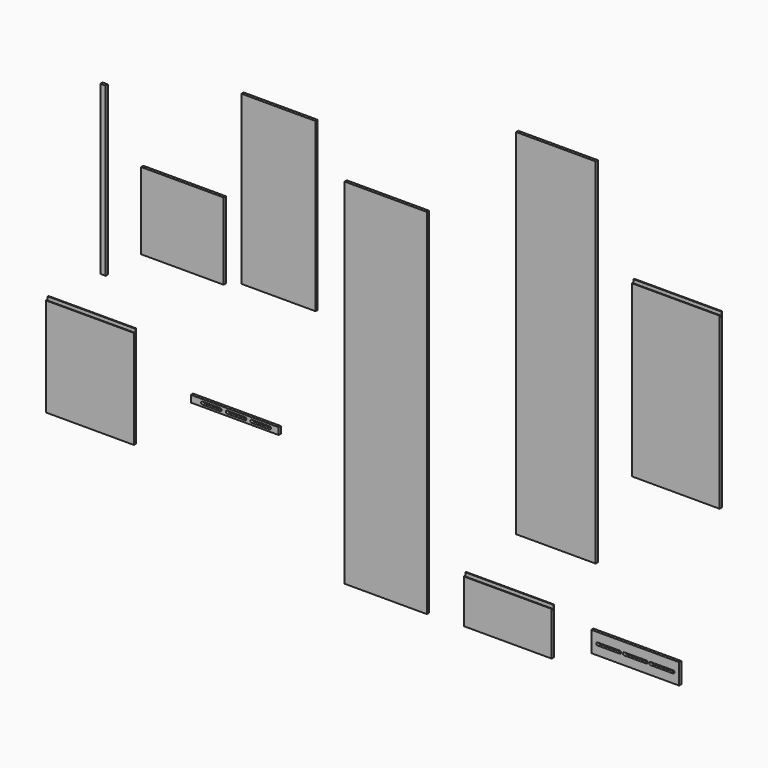
from build123d import *

# Parameters (mm, degrees)
F0_W      = 60
F0_H      = 258
F1_DEPTH  = 2
F2_W      = 58
F2_H      = 258
F3_DEPTH  = 2
F4_W      = 60
F4_H      = 56
F5_DEPTH  = 2
F6_W      = 64
F6_H      = 5
F7_DEPTH  = 2
F8_W      = 64
F8_H      = 74
F9_DEPTH  = 2
F10_W     = 64
F10_H     = 15
F11_DEPTH = 2
F13_DEPTH = 4
F14_W     = 64
F14_H     = 126
F15_DEPTH = 2
F16_W     = 64
F16_H     = 34
F17_DEPTH = 2
F18_W     = 54
F18_H     = 122
F19_DEPTH = 2
F20_W     = 4
F20_H     = 122
F21_DEPTH = 2
F23_DEPTH = 64
F24_R     = 0.2
F26_DEPTH = 64
F27_R     = 0.2
F29_DEPTH = 64
F30_R     = 0.2


with BuildPart() as f1:
    # F0 (on Front) → F1 (new body)
    with BuildSketch(Plane.XZ):
        with Locations((-45.8140162975, 94.1403650641)):
            Rectangle(F0_W, F0_H)
    extrude(amount=F1_DEPTH)


with BuildPart() as f3:
    # F2 (on Front) → F3 (new body)
    with BuildSketch(Plane.XZ):
        with Locations((78.1819216013, 166.5537835062)):
            Rectangle(F2_W, F2_H)
    extrude(amount=F3_DEPTH)


with BuildPart() as f5:
    # F4 (on Front) → F5 (new body)
    with BuildSketch(Plane.XZ):
        with Locations((-193.9391981363, 156.2652424913)):
            Rectangle(F4_W, F4_H)
    extrude(amount=F5_DEPTH)


with BuildPart() as f7:
    # F6 (on Front) → F7 (new body)
    with BuildSketch(Plane.XZ):
        with Locations((-155.7672946453, 47.4037402868)):
            Rectangle(F6_W, F6_H)
        with BuildLine():
            ThreePointArc((-180.3556742668, 47.3932959139), (-180.062781048, 48.1004026951), (-179.3556742668, 48.3932959139))
            Line((-179.3556742668, 48.3932959139), (-166.3556742668, 48.3932959139))
            ThreePointArc((-166.3556742668, 48.3932959139), (-165.6485674856, 48.1004026951), (-165.3556742668, 47.3932959139))
            ThreePointArc((-165.3556742668, 47.3932959139), (-165.6485674856, 46.6861891327), (-166.3556742668, 46.3932959139))
            Line((-166.3556742668, 46.3932959139), (-179.3556742668, 46.3932959139))
            ThreePointArc((-179.3556742668, 46.3932959139), (-180.062781048, 46.6861891327), (-180.3556742668, 47.3932959139))
        make_face(mode=Mode.SUBTRACT)
        with BuildLine():
            ThreePointArc((-162.3556742668, 47.3932959139), (-162.062781048, 48.1004026951), (-161.3556742668, 48.3932959139))
            Line((-161.3556742668, 48.3932959139), (-148.3556742668, 48.3932959139))
            ThreePointArc((-148.3556742668, 48.3932959139), (-147.6485674856, 48.1004026951), (-147.3556742668, 47.3932959139))
            ThreePointArc((-147.3556742668, 47.3932959139), (-147.6485674856, 46.6861891327), (-148.3556742668, 46.3932959139))
            Line((-148.3556742668, 46.3932959139), (-161.3556742668, 46.3932959139))
            ThreePointArc((-161.3556742668, 46.3932959139), (-162.062781048, 46.6861891327), (-162.3556742668, 47.3932959139))
        make_face(mode=Mode.SUBTRACT)
        with BuildLine():
            ThreePointArc((-144.3556742668, 47.3932959139), (-144.062781048, 48.1004026951), (-143.3556742668, 48.3932959139))
            Line((-143.3556742668, 48.3932959139), (-130.3556742668, 48.3932959139))
            ThreePointArc((-130.3556742668, 48.3932959139), (-129.6485674856, 48.1004026951), (-129.3556742668, 47.3932959139))
            ThreePointArc((-129.3556742668, 47.3932959139), (-129.6485674856, 46.6861891327), (-130.3556742668, 46.3932959139))
            Line((-130.3556742668, 46.3932959139), (-143.3556742668, 46.3932959139))
            ThreePointArc((-143.3556742668, 46.3932959139), (-144.062781048, 46.6861891327), (-144.3556742668, 47.3932959139))
        make_face(mode=Mode.SUBTRACT)
    extrude(amount=F7_DEPTH)


with BuildPart() as f9:
    # F8 (on Front) → F9 (new body)
    with BuildSketch(Plane.XZ):
        with Locations((-261.2743257284, 41.2309435084)):
            Rectangle(F8_W, F8_H)
    extrude(amount=F9_DEPTH)

    # F22 (on face) → F23 (cut)
    with BuildSketch(Plane.YZ.offset(-229.2743257284)):
        with BuildLine():
            Line((-0.5, 78.2309435084), (-2, 78.2309435084))
            Line((-2, 78.2309435084), (-2, 76.2309435084))
            Line((-2, 76.2309435084), (-1.5, 76.2309435084))
            Line((-1.5, 76.2309435084), (-1.5, 75.7309435084))
            ThreePointArc((-1.5, 75.7309435084), (-1.2071067812, 75.0238367273), (-0.5, 74.7309435084))
            Line((-0.5, 74.7309435084), (-0.5, 78.2309435084))
        make_face()
    extrude(amount=-F23_DEPTH, mode=Mode.SUBTRACT)

    # F24
    f24_edges = [f9.edges().sort_by_distance(p)[0] for p in [
        (-261.274326, -0.5, 78.230944),
        (-261.274326, -2, 76.230944),
        (-261.274326, -0.5, 74.730944),
        (-261.274326, -1.5, 76.230944),
    ]]
    fillet(f24_edges, radius=F24_R)


with BuildPart() as f11:
    # F10 (on Front) → F11 (new body)
    with BuildSketch(Plane.XZ):
        with Locations((136.0173345804, -13.4328569472)):
            Rectangle(F10_W, F10_H)
    extrude(amount=F11_DEPTH)

    # F12 (on Front) → F13 (cut)
    with BuildSketch(Plane.XZ):
        with BuildLine():
            Line((124.9154765659, -12.5541486777), (108.4641042895, -12.5541486777))
            ThreePointArc((108.4641042895, -12.5541486777), (107.916581707, -12.7809399571), (107.6897904277, -13.3284625395))
            Line((107.6897904277, -13.3284625395), (107.6897904277, -13.7798348159))
            ThreePointArc((107.6897904277, -13.7798348159), (107.916581707, -14.3273573984), (108.4641042895, -14.5541486777))
            Line((108.4641042895, -14.5541486777), (124.9154765659, -14.5541486777))
            ThreePointArc((124.9154765659, -14.5541486777), (125.4629991483, -14.3273573984), (125.6897904277, -13.7798348159))
            Line((125.6897904277, -13.7798348159), (125.6897904277, -13.3284625395))
            ThreePointArc((125.6897904277, -13.3284625395), (125.4629991483, -12.7809399571), (124.9154765659, -12.5541486777))
        make_face()
        with BuildLine():
            Line((144.3154765659, -12.5541477464), (127.8641042895, -12.5541477464))
            ThreePointArc((127.8641042895, -12.5541477464), (127.316581707, -12.7809390258), (127.0897904277, -13.3284616082))
            Line((127.0897904277, -13.3284616082), (127.0897904277, -13.7798348159))
            ThreePointArc((127.0897904277, -13.7798348159), (127.316581707, -14.3273573984), (127.8641042895, -14.5541486777))
            Line((127.8641042895, -14.5541486777), (144.3154765659, -14.5541486777))
            ThreePointArc((144.3154765659, -14.5541486777), (144.8629991483, -14.3273573984), (145.0897904277, -13.7798348159))
            Line((145.0897904277, -13.7798348159), (145.0897904277, -13.3284616082))
            ThreePointArc((145.0897904277, -13.3284616082), (144.8629991483, -12.7809390258), (144.3154765659, -12.5541477464))
        make_face()
        with BuildLine():
            Line((163.7154765659, -12.5129134394), (147.2641042895, -12.5129134394))
            ThreePointArc((147.2641042895, -12.5129134394), (146.716581707, -12.7397047188), (146.4897904277, -13.2872273012))
            Line((146.4897904277, -13.2872273012), (146.4897904277, -13.8210691229))
            ThreePointArc((146.4897904277, -13.8210691229), (146.716581707, -14.3685917054), (147.2641042895, -14.5953829847))
            Line((147.2641042895, -14.5953829847), (163.7154765659, -14.5953829847))
            ThreePointArc((163.7154765659, -14.5953829847), (164.2629991483, -14.3685917054), (164.4897904277, -13.8210691229))
            Line((164.4897904277, -13.8210691229), (164.4897904277, -13.2872273012))
            ThreePointArc((164.4897904277, -13.2872273012), (164.2629991483, -12.7397047188), (163.7154765659, -12.5129134394))
        make_face()
    extrude(amount=F13_DEPTH, mode=Mode.SUBTRACT)


with BuildPart() as f15:
    # F14 (on Front) → F15 (new body)
    with BuildSketch(Plane.XZ):
        with Locations((165.5951834917, 165.0863875747)):
            Rectangle(F14_W, F14_H)
    extrude(amount=F15_DEPTH)

    # F25 (on face) → F26 (cut)
    with BuildSketch(Plane.YZ.offset(197.5951834917)):
        with BuildLine():
            Line((-0.5, 228.0863875747), (-2, 228.0863875747))
            Line((-2, 228.0863875747), (-2, 226.0863875747))
            Line((-2, 226.0863875747), (-1.5, 226.0863875747))
            Line((-1.5, 226.0863875747), (-1.5, 225.5863875747))
            ThreePointArc((-1.5, 225.5863875747), (-1.2071067812, 224.8792807935), (-0.5, 224.5863875747))
            Line((-0.5, 224.5863875747), (-0.5, 228.0863875747))
        make_face()
    extrude(amount=-F26_DEPTH, mode=Mode.SUBTRACT)

    # F27
    f27_edges = [f15.edges().sort_by_distance(p)[0] for p in [
        (165.595183, -0.5, 228.086388),
        (165.595183, -2, 226.086388),
        (165.595183, -1.5, 226.086388),
    ]]
    fillet(f27_edges, radius=F27_R)


with BuildPart() as f17:
    # F16 (on Front) → F17 (new body)
    with BuildSketch(Plane.XZ):
        with Locations((43.1058065668, -16.8282787427)):
            Rectangle(F16_W, F16_H)
    extrude(amount=F17_DEPTH)

    # F28 (on face) → F29 (cut)
    with BuildSketch(Plane.YZ.offset(75.1058065668)):
        with BuildLine():
            Line((-0.5, 0.1717212573), (-2, 0.1717212573))
            Line((-2, 0.1717212573), (-2, -1.8282787427))
            Line((-2, -1.8282787427), (-1.5, -1.8282787427))
            Line((-1.5, -1.8282787427), (-1.5, -2.3282787427))
            ThreePointArc((-1.5, -2.3282787427), (-1.2071067812, -3.0353855239), (-0.5, -3.3282787427))
            Line((-0.5, -3.3282787427), (-0.5, 0.1717212573))
        make_face()
    extrude(amount=-F29_DEPTH, mode=Mode.SUBTRACT)

    # F30
    f30_edges = [f17.edges().sort_by_distance(p)[0] for p in [
        (43.105807, -0.5, 0.171721),
        (43.105807, -1.5, -1.828279),
        (43.105807, -2, -1.828279),
    ]]
    fillet(f30_edges, radius=F30_R)


with BuildPart() as f19:
    # F18 (on Front) → F19 (new body)
    with BuildSketch(Plane.XZ):
        with Locations((-123.9371697903, 194.0556869507)):
            Rectangle(F18_W, F18_H)
    extrude(amount=F19_DEPTH)


with BuildPart() as f21:
    # F20 (on Front) → F21 (new body)
    with BuildSketch(Plane.XZ):
        with Locations((-251.7955411673, 167.0450652838)):
            Rectangle(F20_W, F20_H)
    extrude(amount=F21_DEPTH)


solid = Compound([f1.part, f3.part, f5.part, f7.part, f9.part, f11.part, f15.part, f17.part, f19.part, f21.part])
